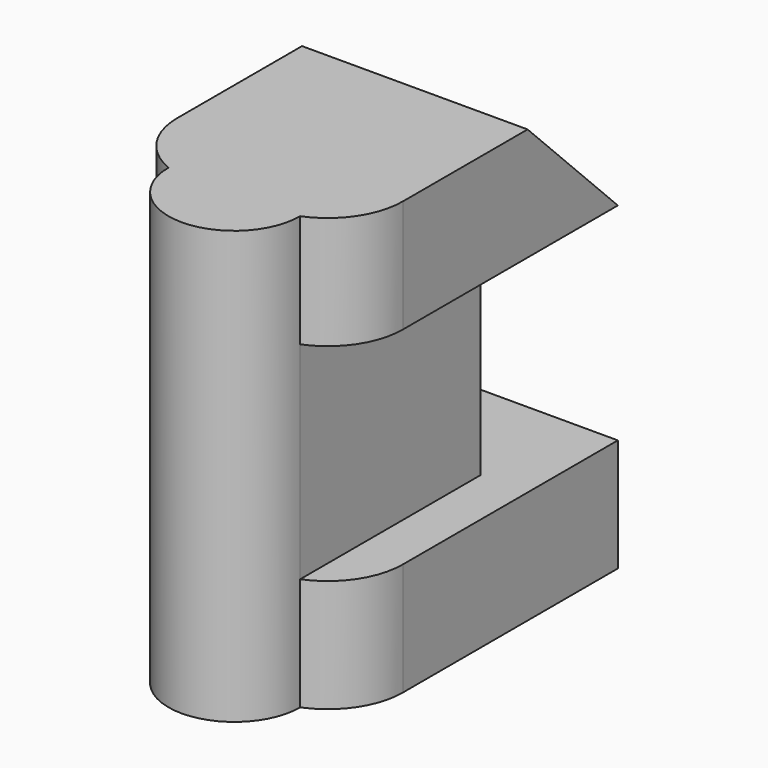
from build123d import *

# Parameters (mm, degrees)
F0_W        = 3.5
F0_H        = 5.5
F1_DEPTH    = 6
F2_W        = 1.75
F2_H        = 11.5
F4_T1_DEPTH = 12.2702481089
F4_T3_DEPTH = 12.2702481089
F5_W        = 6
F5_H        = 3
F6_DEPTH    = 3
F8_DEPTH    = 25


# Not quite as in the source:
# - a fillet or chamfer that OpenCascade refuses, or shapes differently, is made with other operations: its cross-section is extruded or revolved along the edge and cut away or added


with BuildPart() as f1:
    # F0 (on Front) → F1 (new body)
    with BuildSketch(Plane.XZ):
        Polygon((1.75, -1.5), (3, -1.5), (3, 1.5), (-3, 1.5), (-3, -1.5), (-1.75, -1.5), align=None)
        with Locations((0, -4.25)):
            Rectangle(F0_W, F0_H)
        Polygon((3, -7), (1.75, -7), (-1.75, -7), (-3, -7), (-3, -10), (3, -10), align=None)
    extrude(amount=F1_DEPTH)

    # F2 (on face) → F3 (revolve)
    with BuildSketch(Plane.XZ.offset(6)):
        with Locations((-0.875, -4.25)):
            Rectangle(F2_W, F2_H)
    revolve(axis=Axis((0, -6, -4.25), (0, 0, -1)))

    # F4: fillet of radius 2 on 4 edges, made by hand

    # F4_s2 → F4_t1 (cut)
    with BuildSketch(Plane.XY.offset(-6.1351240544)):
        with BuildLine():
            ThreePointArc((3, -4.1459503782), (2.6583123952, -5.263984367), (1.75, -6))
            Line((1.75, -6), (3, -6))
            Line((3, -6), (3, -4.1459503782))
        make_face()
        with BuildLine():
            ThreePointArc((-3, -4.1459503782), (-2.6583123952, -5.263984367), (-1.75, -6))
            Line((-1.75, -6), (-3, -6))
            Line((-3, -6), (-3, -4.1459503782))
        make_face()
    extrude(amount=F4_T1_DEPTH, mode=Mode.SUBTRACT)

    # F4_s4 → F4_t3 (cut)
    with BuildSketch(Plane.XY.offset(-14.6351240544)):
        with BuildLine():
            ThreePointArc((3, -4.1459503782), (2.6583123952, -5.263984367), (1.75, -6))
            Line((1.75, -6), (3, -6))
            Line((3, -6), (3, -4.1459503782))
        make_face()
        with BuildLine():
            ThreePointArc((-3, -4.1459503782), (-2.6583123952, -5.263984367), (-1.75, -6))
            Line((-1.75, -6), (-3, -6))
            Line((-3, -6), (-3, -4.1459503782))
        make_face()
    extrude(amount=F4_T3_DEPTH, mode=Mode.SUBTRACT)

    # F5 (on face) → F6 (join)
    with BuildSketch(Plane(origin=(0, 0, 0), x_dir=(-1, 0, 0), z_dir=(0, 1, 0))):
        Rectangle(F5_W, F5_H)
        with Locations((0, -8.5)):
            Rectangle(F5_W, F5_H)
    extrude(amount=F6_DEPTH)

    # F7 (on face) → F8 (cut)
    with BuildSketch(Plane.YZ.offset(3)):
        Polygon((0, 1.5), (3, -1.5), (3, 1.5), align=None)
    extrude(amount=-F8_DEPTH, mode=Mode.SUBTRACT)


solid = f1.part
